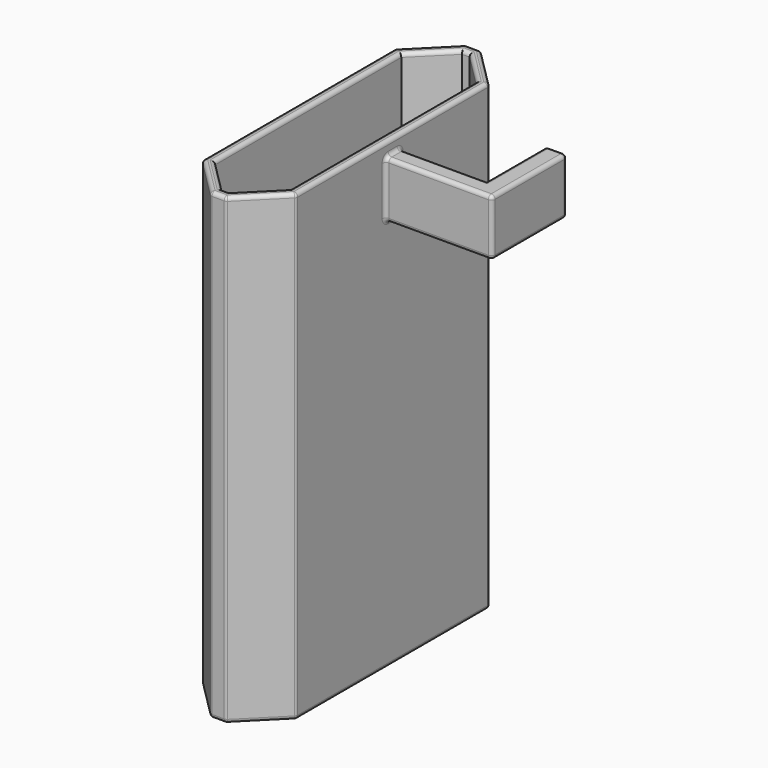
from build123d import *

# Parameters (mm, degrees)
F1_DEPTH = 2.5
F2_DEPTH = 123.5
F3_W     = 5
F3_H     = 15
F4_DEPTH = 28.5
F5_START = 23
F3_W_2   = 20
F5_DEPTH = 5.5
F6_R     = 1


with BuildPart() as f1:
    # F0 (on Top) → F1 (new body)
    with BuildSketch(Plane.XY):
        Polygon((10, 31), (1, 40), (-1, 40), (-10, 31), (-10, -31), (-1, -40), (1, -40), (10, -31), align=None)
    extrude(amount=F1_DEPTH)

    # F0 (on Top) → F2 (join)
    with BuildSketch(Plane.XY):
        Polygon((12.500000447, -32.0355340911), (12.500000447, 32.0355340911), (2.0355340911, 42.500000447), (-2.0355340911, 42.500000447), (-12.500000447, 32.0355340911), (-12.500000447, -32.0355340911), (-2.0355340911, -42.500000447), (2.0355340911, -42.500000447), align=None)
        Polygon((-1, 40), (1, 40), (10, 31), (10, -31), (1, -40), (-1, -40), (-10, -31), (-10, 31), align=None, mode=Mode.SUBTRACT)
    extrude(amount=F2_DEPTH)

    # F3 (on face) → F4 (join)
    with BuildSketch(Plane.YZ.offset(12.500000447)):
        with Locations((-4.47e-07, 112.5)):
            Rectangle(F3_W, F3_H)
    extrude(amount=F4_DEPTH)

    # F3 (on face) → F5 (join)
    with BuildSketch(Plane.YZ.offset(12.500000447).offset(F5_START)):
        with Locations((12.499999553, 112.5)):
            Rectangle(F3_W_2, F3_H)
    extrude(amount=F5_DEPTH)

    # F6
    f6_edges = [f1.edges().sort_by_distance(p)[0] for p in [
        (12.5, 0, 123.5),
        (7.267767, 37.267767, 123.5),
        (0, 42.5, 123.5),
        (-7.267767, 37.267767, 123.5),
        (-12.5, 0, 123.5),
        (-7.267767, -37.267767, 123.5),
        (0, -42.5, 123.5),
        (7.267767, -37.267767, 123.5),
        (0, 40, 123.5),
        (5.5, 35.5, 123.5),
        (10, 0, 123.5),
        (5.5, -35.5, 123.5),
        (0, -40, 123.5),
        (-5.5, -35.5, 123.5),
        (-10, 0, 123.5),
        (-5.5, 35.5, 123.5),
        (24, 2.5, 120),
        (35.5, 12.5, 120),
        (38.25, 22.5, 120),
        (41, 10, 120),
        (26.75, -2.5, 120),
        (12.5, 0, 120),
        (26.75, -2.5, 105),
        (41, 10, 105),
        (38.25, 22.5, 105),
        (35.5, 12.5, 105),
        (24, 2.5, 105),
        (12.5, 0, 105),
        (12.5, 0, 0),
        (7.267767, 37.267767, 0),
        (0, 42.5, 0),
        (-7.267767, 37.267767, 0),
        (-12.5, 0, 0),
        (-7.267767, -37.267767, 0),
        (0, -42.5, 0),
        (7.267767, -37.267767, 0),
        (-2.035534, 42.5, 61.75),
        (-12.5, 32.035534, 61.75),
        (-12.5, -32.035534, 61.75),
        (-2.035534, -42.5, 61.75),
        (2.035534, 42.5, 61.75),
        (12.5, 32.035534, 61.75),
        (12.5, -32.035534, 61.75),
        (2.035534, -42.5, 61.75),
        (35.5, 22.5, 112.5),
        (41, 22.5, 112.5),
        (41, -2.5, 112.5),
        (12.5, 2.5, 112.5),
        (12.5, -2.5, 112.5),
    ]]
    fillet(f6_edges, radius=F6_R)


solid = f1.part
